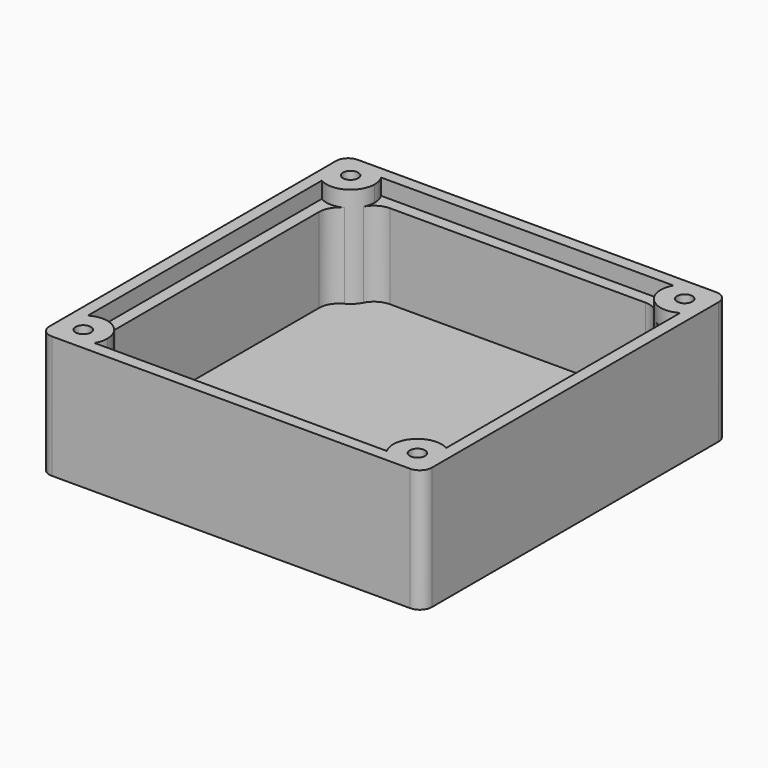
from build123d import *

# Parameters (mm, degrees)
F0_W        = 95
F0_H        = 95
F1_DEPTH    = 30.5
F3_DEPTH    = 25
F4_R        = 1.9
F5_DEPTH    = 30.501
F6_R        = 3
F7_W        = 72.6076951546
F7_H        = 3
F7_W_2      = 3
F7_H_2      = 72.6076951546
F8_DEPTH    = 21
F9_T1_DEPTH = 21
F10_R       = 3.5
F11_DEPTH   = 15.5


# Not quite as in the source:
# - a fillet or chamfer that OpenCascade refuses, or shapes differently, is made with other operations: its cross-section is extruded or revolved along the edge and cut away or added


with BuildPart() as f1:
    # F0 (on Top) → F1 (new body)
    with BuildSketch(Plane.XY):
        Rectangle(F0_W, F0_H)
    extrude(amount=F1_DEPTH)

    # F2 (on face) → F3 (cut)
    with BuildSketch(Plane.XY.offset(30.5)):
        with BuildLine():
            Line((36.3038475773, 44.5), (-36.3038475773, 44.5))
            ThreePointArc((-36.3038475773, 44.5), (-35.7044450423, 43.0529142706), (-35.5, 41.5))
            ThreePointArc((-35.5, 41.5), (-38.5, 36.3038475773), (-44.5, 36.3038475773))
            Line((-44.5, 36.3038475773), (-44.5, -36.3038475773))
            ThreePointArc((-44.5, -36.3038475773), (-38.5, -36.3038475773), (-35.5, -41.5))
            ThreePointArc((-35.5, -41.5), (-35.7044450423, -43.0529142706), (-36.3038475773, -44.5))
            Line((-36.3038475773, -44.5), (36.3038475773, -44.5))
            ThreePointArc((36.3038475773, -44.5), (37.2573593129, -37.2573593129), (44.5, -36.3038475773))
            Line((44.5, -36.3038475773), (44.5, 36.3038475773))
            ThreePointArc((44.5, 36.3038475773), (37.2573593129, 37.2573593129), (36.3038475773, 44.5))
        make_face()
    extrude(amount=-F3_DEPTH, mode=Mode.SUBTRACT)

    # F4 (on face) → F5 (cut, through all)
    with BuildSketch(Plane.XY.offset(30.5)):
        with Locations((-41.5, 41.5)):
            Circle(F4_R)
        with Locations((41.5, 41.5)):
            Circle(F4_R)
        with Locations((-41.5, -41.5)):
            Circle(F4_R)
        with Locations((41.5, -41.5)):
            Circle(F4_R)
    extrude(amount=-F5_DEPTH, mode=Mode.SUBTRACT)

    # F6
    f6_edges = [f1.edges().sort_by_distance(p)[0] for p in [
        (-47.5, 47.5, 15.25),
        (47.5, 47.5, 15.25),
        (-47.5, -47.5, 15.25),
        (47.5, -47.5, 15.25),
    ]]
    fillet(f6_edges, radius=F6_R)

    # F7 (on face) → F8 (join)
    with BuildSketch(Plane.XY.offset(5.5)):
        with Locations((0, 43)):
            Rectangle(F7_W, F7_H)
        with Locations((-43, 0)):
            Rectangle(F7_W_2, F7_H_2)
        with Locations((0, -43)):
            Rectangle(F7_W, F7_H)
        with Locations((43, 0)):
            Rectangle(F7_W_2, F7_H_2)
    extrude(amount=F8_DEPTH)

    # F9: fillet of radius 5 on 8 edges, made by hand

    # F9_s2 → F9_t1 (join)
    with BuildSketch(Plane.XY.offset(5.5)):
        with BuildLine():
            ThreePointArc((-36.155658743, 38.7727272727), (-34.3132058682, 40.7640143271), (-31.7020410289, 41.5))
            Line((-31.7020410289, 41.5), (-35.5, 41.5))
            ThreePointArc((-35.5, 41.5), (-35.6662170274, 40.0975107027), (-36.155658743, 38.7727272727))
        make_face()
        with BuildLine():
            ThreePointArc((-38.7727272727, 36.155658743), (-40.7640143271, 34.3132058682), (-41.5, 31.7020410289))
            Line((-41.5, 31.7020410289), (-41.5, 35.5))
            ThreePointArc((-41.5, 35.5), (-40.0975107027, 35.6662170274), (-38.7727272727, 36.155658743))
        make_face()
        with BuildLine():
            ThreePointArc((36.155658743, 38.7727272727), (34.3132058682, 40.7640143271), (31.7020410289, 41.5))
            Line((31.7020410289, 41.5), (35.5, 41.5))
            ThreePointArc((35.5, 41.5), (35.6662170274, 40.0975107027), (36.155658743, 38.7727272727))
        make_face()
        with BuildLine():
            ThreePointArc((38.7727272727, 36.155658743), (40.7640143271, 34.3132058682), (41.5, 31.7020410289))
            Line((41.5, 31.7020410289), (41.5, 35.5))
            ThreePointArc((41.5, 35.5), (40.0975107027, 35.6662170274), (38.7727272727, 36.155658743))
        make_face()
        with BuildLine():
            ThreePointArc((38.7727272727, -36.155658743), (40.7640143271, -34.3132058682), (41.5, -31.7020410289))
            Line((41.5, -31.7020410289), (41.5, -35.5))
            ThreePointArc((41.5, -35.5), (40.0975107027, -35.6662170274), (38.7727272727, -36.155658743))
        make_face()
        with BuildLine():
            ThreePointArc((36.155658743, -38.7727272727), (34.3132058682, -40.7640143271), (31.7020410289, -41.5))
            Line((31.7020410289, -41.5), (35.5, -41.5))
            ThreePointArc((35.5, -41.5), (35.6662170274, -40.0975107027), (36.155658743, -38.7727272727))
        make_face()
        with BuildLine():
            ThreePointArc((-38.7727272727, -36.155658743), (-40.7640143271, -34.3132058682), (-41.5, -31.7020410289))
            Line((-41.5, -31.7020410289), (-41.5, -35.5))
            ThreePointArc((-41.5, -35.5), (-40.0975107027, -35.6662170274), (-38.7727272727, -36.155658743))
        make_face()
        with BuildLine():
            ThreePointArc((-36.155658743, -38.7727272727), (-34.3132058682, -40.7640143271), (-31.7020410289, -41.5))
            Line((-31.7020410289, -41.5), (-35.5, -41.5))
            ThreePointArc((-35.5, -41.5), (-35.6662170274, -40.0975107027), (-36.155658743, -38.7727272727))
        make_face()
    extrude(amount=F9_T1_DEPTH)

    # F10 (on face) → F11 (cut)
    with BuildSketch(Plane(origin=(0, 0, 0), x_dir=(1, 0, 0), z_dir=(0, 0, -1))):
        with Locations((-41.5, 41.5)):
            Circle(F10_R)
        with Locations((41.5, 41.5)):
            Circle(F10_R)
        with Locations((-41.5, -41.5)):
            Circle(F10_R)
        with Locations((41.5, -41.5)):
            Circle(F10_R)
    extrude(amount=-F11_DEPTH, mode=Mode.SUBTRACT)


solid = f1.part
